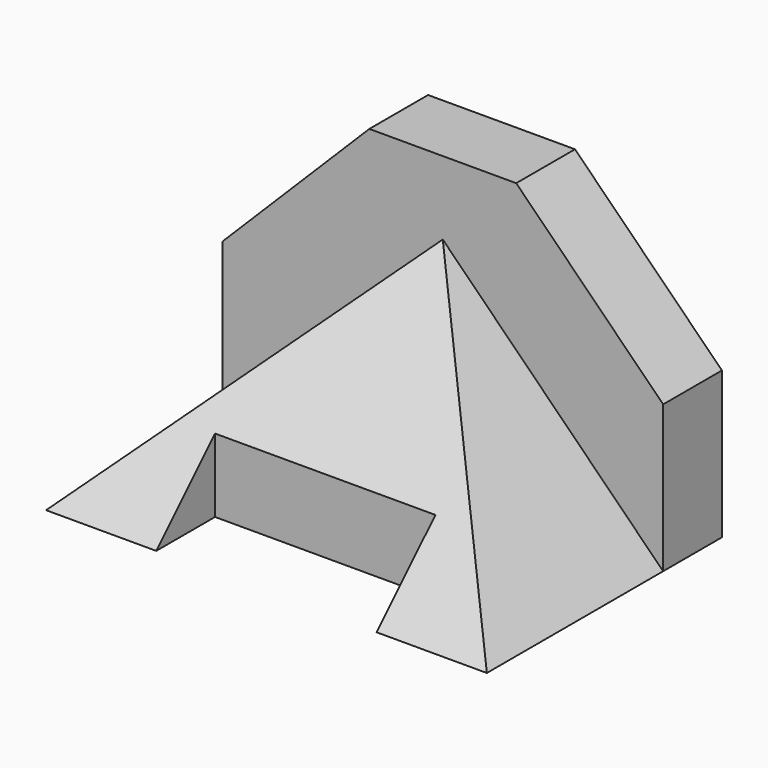
from build123d import *

# Parameters (mm, degrees)
F0_W          = 25.4
F0_H          = 12.7
F1_DEPTH      = 50.8
F2_DEPTH      = 38.1
F4_DEPTH      = 50.801
F5_DEPTH      = 38.1
F7_DEPTH      = 12.7
F9_DEPTH      = 38.101
F9_DEPTH_BACK = 38.101


with BuildPart() as f1:
    # F0 (on Top) → F1 (new body)
    with BuildSketch(Plane.XY):
        with Locations((-25.4, 44.45)):
            Rectangle(F0_W, F0_H)
        Polygon((12.7, 50.8), (-12.7, 50.8), (-12.7, 38.1), (0, 38.1), (12.7, 38.1), align=None)
        with Locations((25.4, 44.45)):
            Rectangle(F0_W, F0_H)
    extrude(amount=F1_DEPTH)

    # F0 (on Top) → F2 (join)
    with BuildSketch(Plane.XY):
        Polygon((0, 38.1), (-38.1, 0), (-19.05, 0), (-19.05, 12.7), (19.05, 12.7), (19.05, 0), (38.1, 0), align=None)
        Polygon((12.7, 38.1), (0, 38.1), (38.1, 0), (38.1, 38.1), align=None)
        Polygon((-12.7, 38.1), (-38.1, 38.1), (-38.1, 0), (0, 38.1), align=None)
    extrude(amount=F2_DEPTH)

    # F3 (on Front) → F4 (cut, through all)
    with BuildSketch(Plane.XZ):
        Polygon((-38.1, 38.1), (-38.1, 25.4), (-25.4, 38.1), align=None)
        Polygon((-38.1, 50.8), (-38.1, 38.1), (-25.4, 38.1), (-12.7, 50.8), align=None)
        Polygon((25.4, 38.1), (38.1, 25.4), (38.1, 38.1), align=None)
        Polygon((38.1, 50.8), (12.7, 50.8), (25.4, 38.1), (38.1, 38.1), align=None)
    extrude(amount=-F4_DEPTH, mode=Mode.SUBTRACT)

    # F3 (on Front) → F5 (cut, through all)
    with BuildSketch(Plane.XZ):
        Polygon((-38.1, 25.4), (-38.1, 0), (-19.05, 19.05), (-19.05, 38.1), (-25.4, 38.1), align=None)
        Polygon((-19.05, 38.1), (-19.05, 19.05), (0, 38.1), align=None)
        Polygon((19.05, 38.1), (0, 38.1), (19.05, 19.05), align=None)
        Polygon((19.05, 38.1), (19.05, 19.05), (38.1, 0), (38.1, 25.4), (25.4, 38.1), align=None)
        Polygon((25.4, 38.1), (38.1, 25.4), (38.1, 38.1), align=None)
    extrude(amount=-F5_DEPTH, mode=Mode.SUBTRACT)

    # F6 (on face) → F7 (join, through all)
    with BuildSketch(Plane.XZ.offset(-12.7)):
        Polygon((-19.05, 12.7), (19.05, 12.7), (19.05, 19.05), (0, 38.1), (-19.05, 19.05), align=None)
    extrude(amount=F7_DEPTH)

    # F8 (on Right) → F9 (cut, two sides)
    with BuildSketch(Plane.YZ) as f9_sk:
        Polygon((0, 0), (38.1, 38.1), (7e-10, 38.1), align=None)
    extrude(amount=-F9_DEPTH, mode=Mode.SUBTRACT)
    extrude(f9_sk.sketch, amount=F9_DEPTH_BACK, mode=Mode.SUBTRACT)


solid = f1.part
